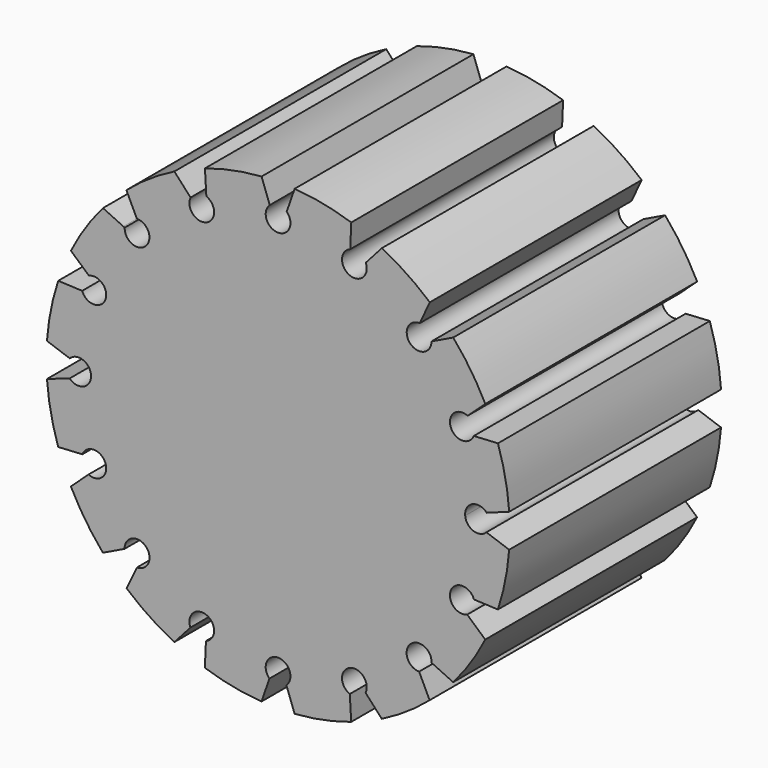
from build123d import *

# Parameters (mm, degrees)
F1_DEPTH = 20


# Not quite as in the source:
# - ends of sketch curves that miss each other by under 0.0002 mm in the source are joined


with BuildPart() as f1:
    # F0 (on Front) → F1 (new body, symmetric)
    with BuildSketch(Plane.XZ):
        with BuildLine():
            Line((34.9101450984, 2.4936542119), (34.9110309298, 2.4939766282))
            ThreePointArc((34.9110309298, 2.4939766282), (34.3286939173, 6.8220798831), (33.2119055423, 11.0439725756))
            Line((33.2119055423, 11.0439725756), (29.5663055038, 10.8358313755))
            ThreePointArc((29.5663055038, 10.8358313755), (26.0913542461, 10.8432258269), (28.6289762641, 13.2172130666))
            Line((28.6289762641, 13.2172130666), (31.2984883804, 15.6633702382))
            Line((31.2984883804, 15.6633702382), (31.2991833986, 15.6640071049))
            ThreePointArc((31.2991833986, 15.6640071049), (29.1048807425, 19.4398023901), (26.457454434, 22.9129462285))
            Line((26.457454434, 22.9129462285), (23.1690113636, 21.3255380981))
            ThreePointArc((23.1690113636, 21.3255380981), (19.9557452862, 20.0025634058), (21.3917167446, 23.1669475309))
            Line((21.3917167446, 23.1669475309), (22.9219205281, 26.4484801345))
            Line((22.9219205281, 26.4484801345), (22.9223189227, 26.4493344946))
            ThreePointArc((22.9223189227, 26.4493344946), (19.450113311, 29.0979912054), (15.6750957256, 31.2936315245))
            Line((15.6750957256, 31.2936315245), (13.2444452709, 28.5686249618))
            ThreePointArc((13.2444452709, 28.5686249618), (10.7820550057, 26.1166920299), (10.897762267, 29.5897242426))
            Line((10.897762267, 29.5897242426), (11.055698063, 33.2070486864))
            Line((11.055698063, 33.2070486864), (11.0557391823, 33.2079904712))
            ThreePointArc((11.0557391823, 33.2079904712), (6.8342424437, 34.3262746336), (2.5063457881, 34.9101450984))
            Line((2.5063457881, 34.9101450984), (1.3035324469, 31.4623976502))
            ThreePointArc((1.3035324469, 31.4623976502), (-0.0331054099, 28.2547910408), (-1.2552777272, 31.5077336698))
            Line((-1.2552777272, 31.5077336698), (-2.4936542119, 34.9101450984))
            Line((-2.4936542119, 34.9101450984), (-2.4939766282, 34.9110309298))
            ThreePointArc((-2.4939766282, 34.9110309298), (-6.8220798831, 34.3286939173), (-11.0439725756, 33.2119055423))
            Line((-11.0439725756, 33.2119055423), (-10.8358313755, 29.5663055038))
            ThreePointArc((-10.8358313755, 29.5663055038), (-10.8432258269, 26.0913542461), (-13.2172130666, 28.6289762641))
            Line((-13.2172130666, 28.6289762641), (-15.6633702382, 31.2984883804))
            Line((-15.6633702382, 31.2984883804), (-15.6640071049, 31.2991833986))
            ThreePointArc((-15.6640071049, 31.2991833986), (-19.4398023901, 29.1048807425), (-22.9129462285, 26.457454434))
            Line((-22.9129462285, 26.457454434), (-21.3255380981, 23.1690113636))
            ThreePointArc((-21.3255380981, 23.1690113636), (-20.0014808321, 19.9567910089), (-23.1670922293, 21.3887099076))
            Line((-23.1670922293, 21.3887099076), (-23.3543714527, 21.4791139546))
            Line((-23.3543714527, 21.4791139546), (-26.4484801345, 22.9219205281))
            Line((-26.4484801345, 22.9219205281), (-26.4493344946, 22.9223189227))
            ThreePointArc((-26.4493344946, 22.9223189227), (-29.0979912054, 19.450113311), (-31.2936315245, 15.6750957256))
            Line((-31.2936315245, 15.6750957256), (-28.5686249618, 13.2444452709))
            ThreePointArc((-28.5686249618, 13.2444452709), (-26.1166920299, 10.7820550057), (-29.5897242426, 10.897762267))
            Line((-29.5897242426, 10.897762267), (-33.2070486864, 11.055698063))
            Line((-33.2070486864, 11.055698063), (-33.2079904712, 11.0557391823))
            ThreePointArc((-33.2079904712, 11.0557391823), (-34.3262746336, 6.8342424437), (-34.9101450984, 2.5063457881))
            Line((-34.9101450984, 2.5063457881), (-31.4623976502, 1.3035324469))
            ThreePointArc((-31.4623976502, 1.3035324469), (-29.3324543071, 1.6932130885), (-28.2642048894, -0.1902286623))
            ThreePointArc((-28.2642048894, -0.1902286623), (-29.4892446104, -1.8074791131), (-31.4669238904, -1.3547032257))
            Line((-31.4669238904, -1.3547032257), (-34.9066388382, -2.5547142739))
            ThreePointArc((-34.9066388382, -2.5547142739), (-34.3227460841, -6.8519414215), (-33.2119055423, -11.0439725756))
            Line((-33.2119055423, -11.0439725756), (-29.5663055038, -10.8358313755))
            ThreePointArc((-29.5663055038, -10.8358313755), (-26.0913542461, -10.8432258269), (-28.6289762641, -13.2172130666))
            Line((-28.6289762641, -13.2172130666), (-31.2984883804, -15.6633702382))
            Line((-31.2984883804, -15.6633702382), (-31.2991833986, -15.6640071049))
            ThreePointArc((-31.2991833986, -15.6640071049), (-29.1048807425, -19.4398023901), (-26.457454434, -22.9129462285))
            Line((-26.457454434, -22.9129462285), (-23.1867866645, -21.3341186503))
            ThreePointArc((-23.1867866645, -21.3341186503), (-19.9778704256, -19.9570429396), (-21.3046655311, -23.1870732319))
            Line((-21.3046655311, -23.1870732319), (-22.8920736615, -26.4755163023))
            ThreePointArc((-22.8920736615, -26.4755163023), (-19.4334813455, -29.1091017174), (-15.6750957256, -31.2936315245))
            Line((-15.6750957256, -31.2936315245), (-13.2444452709, -28.5686249618))
            ThreePointArc((-13.2444452709, -28.5686249618), (-10.7820550057, -26.1166920299), (-10.897762267, -29.5897242426))
            Line((-10.897762267, -29.5897242426), (-11.055698063, -33.2070486864))
            Line((-11.055698063, -33.2070486864), (-11.0557391823, -33.2079904712))
            ThreePointArc((-11.0557391823, -33.2079904712), (-6.8342424437, -34.3262746336), (-2.5063457881, -34.9101450984))
            Line((-2.5063457881, -34.9101450984), (-1.3035324469, -31.4623976502))
            ThreePointArc((-1.3035324469, -31.4623976502), (-1.3388311966, -28.8194805066), (1.3040932823, -28.7847353157))
            ThreePointArc((1.3040932823, -28.7847353157), (1.8690592706, -30.1571657006), (1.2555114416, -31.5085763676))
            Line((1.2555114416, -31.5085763676), (2.4936542119, -34.9101450984))
            Line((2.4936542119, -34.9101450984), (2.4939766282, -34.9110309298))
            ThreePointArc((2.4939766282, -34.9110309298), (6.8220798831, -34.3286939173), (11.0439725756, -33.2119055423))
            Line((11.0439725756, -33.2119055423), (10.8358313755, -29.5663055038))
            ThreePointArc((10.8358313755, -29.5663055038), (10.8432258269, -26.0913542461), (13.2172130666, -28.6289762641))
            Line((13.2172130666, -28.6289762641), (15.6633702382, -31.2984883804))
            Line((15.6633702382, -31.2984883804), (15.6640071049, -31.2991833986))
            ThreePointArc((15.6640071049, -31.2991833986), (19.4283242222, -29.112543996), (22.8920736615, -26.4755163023))
            Line((22.8920736615, -26.4755163023), (21.3046655311, -23.1870732319))
            ThreePointArc((21.3046655311, -23.1870732319), (19.9999615902, -19.9356459921), (23.1847053682, -21.3955906956))
            Line((23.1847053682, -21.3955906956), (23.6096103837, -21.5981338228))
            Line((23.6096103837, -21.5981338228), (26.4484801345, -22.9219205281))
            Line((26.4484801345, -22.9219205281), (26.4493344946, -22.9223189227))
            ThreePointArc((26.4493344946, -22.9223189227), (29.0979912054, -19.450113311), (31.2936315245, -15.6750957256))
            Line((31.2936315245, -15.6750957256), (28.5686249618, -13.2444452709))
            ThreePointArc((28.5686249618, -13.2444452709), (26.1166920299, -10.7820550057), (29.5897242426, -10.897762267))
            Line((29.5897242426, -10.897762267), (33.2070486864, -11.055698063))
            Line((33.2070486864, -11.055698063), (33.2079904712, -11.0557391823))
            ThreePointArc((33.2079904712, -11.0557391823), (34.3215316909, -6.8580217548), (34.9066388382, -2.5547142739))
            Line((34.9066388382, -2.5547142739), (31.4669238904, -1.3547032257))
            ThreePointArc((31.4669238904, -1.3547032257), (29.4892446104, -1.8074791131), (28.2642048894, -0.1902286623))
            ThreePointArc((28.2642048894, -0.1902286623), (29.3625733997, 1.7069569752), (31.5077336698, 1.2552777272))
            Line((31.5077336698, 1.2552777272), (34.9101450984, 2.4936542119))
        make_face()
    extrude(amount=F1_DEPTH, both=True)


solid = f1.part
